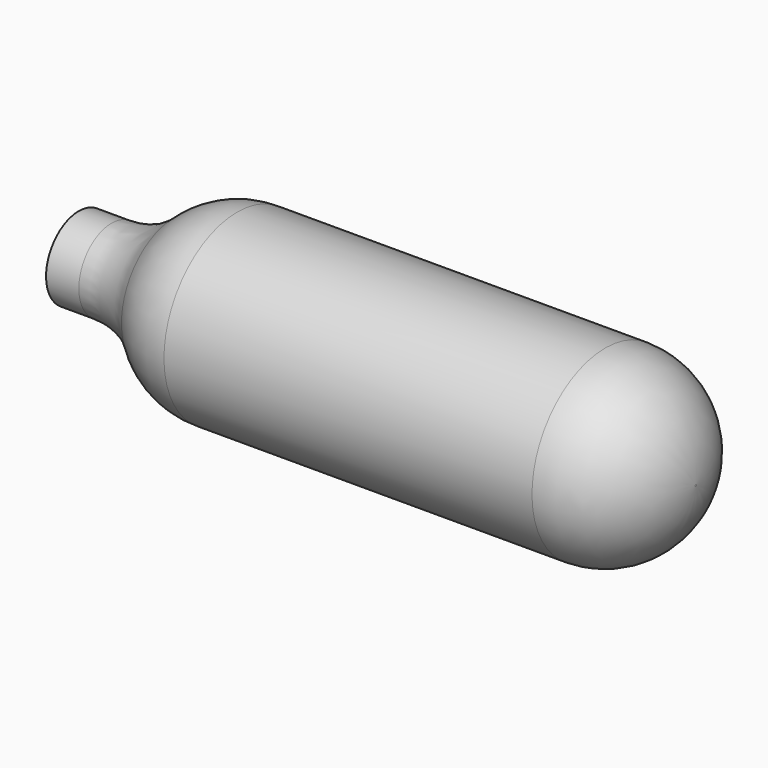
from build123d import *

# Parameters (mm, degrees)
F2_R     = 9.398
F4_R     = 9.398
F5_R     = 0.508
F6_DEPTH = 25.4


# Not quite as in the source:
# - a fillet or chamfer that OpenCascade refuses, or shapes differently, is made with other operations: its cross-section is extruded or revolved along the edge and cut away or added


with BuildPart() as f1:
    # F0 (on Front) → F1 (revolve)
    with BuildSketch(Plane.XZ):
        Polygon((-31.5141436086, 0), (0, 0), (32.4938563914, 0), (32.4938563914, 9.4996), (-23.5131436086, 9.4996), (-23.5131436086, 4.2418), (-31.5141436086, 4.2418), align=None)
    revolve(axis=Axis((16.2469281957, 0, 0), (1, 0, 0)))

    # F2
    f2_edges = [f1.edges().sort_by_distance(p)[0] for p in [
        (32.493856, 0, -9.4996),
    ]]
    fillet(f2_edges, radius=F2_R)

    # F3: fillet of radius 9.398 on 1 edges, made by hand

    # F3_s1 → F3_t2 (revolve, cut)
    with BuildSketch(Plane.XZ):
        with BuildLine():
            ThreePointArc((-15.0762515291, 9.4996), (-20.0468050396, 8.0775640044), (-23.5131436086, 4.2418))
            Line((-23.5131436086, 4.2418), (-23.5131436086, 9.4996))
            Line((-23.5131436086, 9.4996), (-15.0762515291, 9.4996))
        make_face()
    revolve(axis=Axis((-23.5131436086, 0, 0), (1, 0, 0)), mode=Mode.SUBTRACT)

    # F4
    f4_edges = [f1.edges().sort_by_distance(p)[0] for p in [
        (-23.513144, 0, -4.2418),
    ]]
    fillet(f4_edges, radius=F4_R)

    # F5 (on face) → F6 (cut)
    with BuildSketch(Plane(origin=(-31.5141436086, 0, 0), x_dir=(0, -1, 0), z_dir=(-1, 0, 0))):
        Circle(F5_R)
    extrude(amount=-F6_DEPTH, mode=Mode.SUBTRACT)


solid = f1.part
